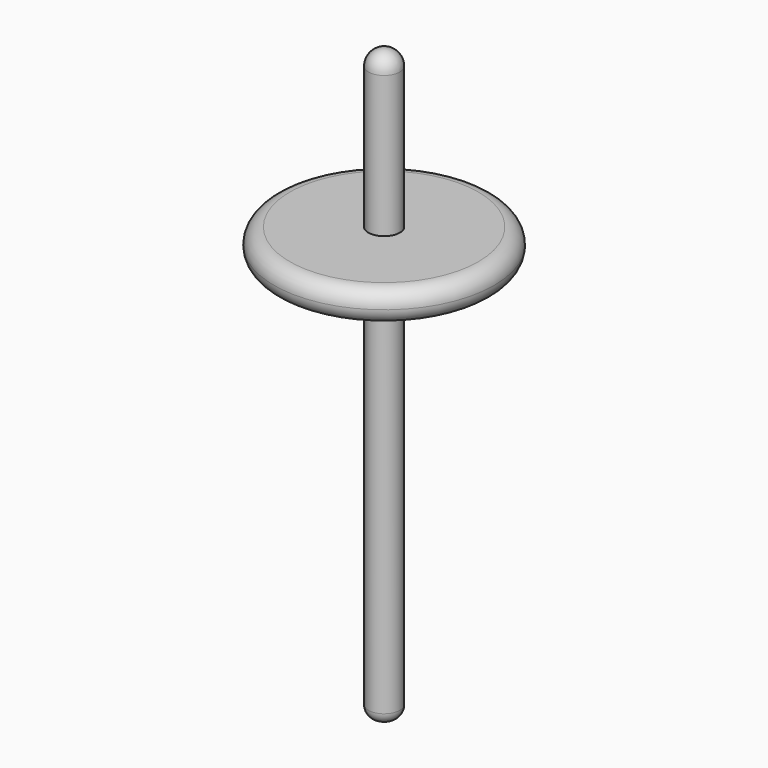
from build123d import *

# Parameters (mm, degrees)
F0_R      = 5.08
F1_DEPTH  = 190.5
F7_R      = 35.56
F8_DEPTH  = 10.16
F9_R      = 5.07999
F11_R     = 7.62
F12_DEPTH = 5.08
F13_R     = 2.53999
F14_R     = 5.08
F16_R     = 3.81


# Not quite as in the source:
# - a fillet or chamfer is up to 0.001 mm smaller than in the source, because OpenCascade refuses the exact size


with BuildPart() as f1:
    # F0 (on Top) → F1 (new body)
    with BuildSketch(Plane.XY):
        Circle(F0_R)
    extrude(amount=F1_DEPTH)

    # F7 (on offset) → F8 (join)
    with BuildSketch(Plane.XY.offset(129.54)):
        Circle(F7_R)
    extrude(amount=F8_DEPTH)

    # F9 (radius 5.08 in the source; OpenCascade refuses exactly that, so slightly less here)
    f9_edges = [f1.edges().sort_by_distance(p)[0] for p in [
        (-35.56, 0, 139.7),
        (-35.56, 0, 129.54),
    ]]
    fillet(f9_edges, radius=F9_R)

    # F14
    f14_edges = [f1.edges().sort_by_distance(p)[0] for p in [
        (-5.08, 0, 190.5),
    ]]
    fillet(f14_edges, radius=F14_R)

    # F16
    f16_edges = [f1.edges().sort_by_distance(p)[0] for p in [
        (-5.08, 0, 0),
    ]]
    fillet(f16_edges, radius=F16_R)


with BuildPart() as f12:
    # F11 (on offset) → F12 (new body)
    with BuildSketch(Plane.XY.offset(193.04)):
        Circle(F11_R)
    extrude(amount=F12_DEPTH)

    # F13 (radius 2.54 in the source; OpenCascade refuses exactly that, so slightly less here)
    f13_edges = [f12.edges().sort_by_distance(p)[0] for p in [
        (-7.62, 0, 193.04),
        (-7.62, 0, 198.12),
    ]]
    fillet(f13_edges, radius=F13_R)


solid = f1.part
